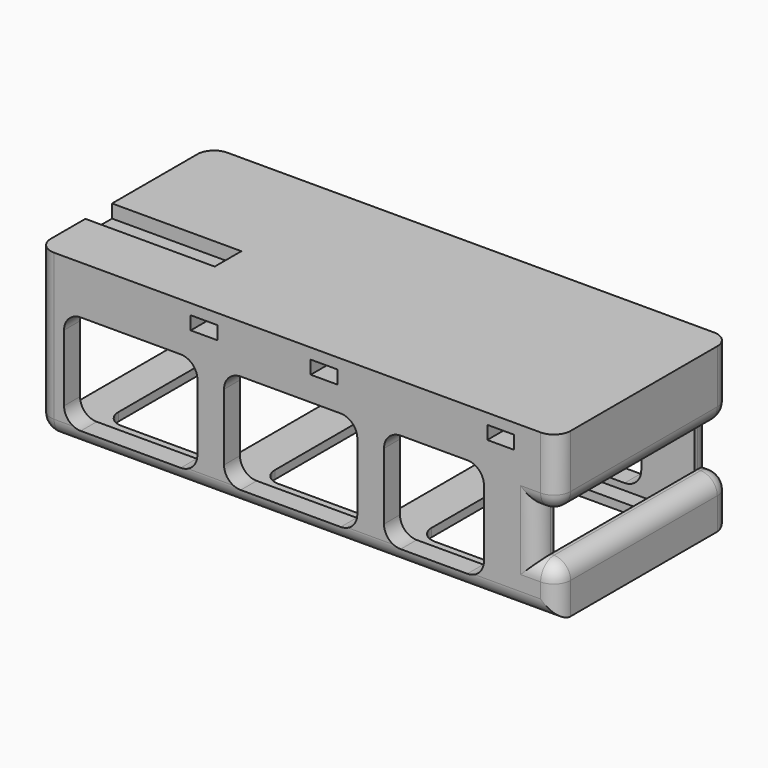
from build123d import *

# Parameters (mm, degrees)
F0_W          = 152
F0_H          = 55
F1_DEPTH      = 39
F2_W          = 53
F2_H          = 34
F3_DEPTH      = 150
F5_DEPTH      = 10.9
F7_DEPTH      = 100
F8_DEPTH      = 5
F9_DEPTH      = 4
F10_DEPTH     = 5
F11_DEPTH     = 5
F12_DEPTH     = 5
F13_W         = 8
F13_H         = 4
F14_DEPTH     = 100
F15_T1_DEPTH  = 163.5
F15_T3_DEPTH  = 74
F15_T5_DEPTH  = 56.5
F15_T7_DEPTH  = 55
F15_S11_W     = 5
F15_S11_H     = 5
F15_T12_DEPTH = 5
F15_S17_W     = 5
F15_S17_H     = 5
F15_T18_DEPTH = 5
F16_W         = 7.2434431314
F16_H         = 13.5
F16_W_2       = 55
F16_W_3       = 10.0454574823
F17_DEPTH     = 6
F18_R         = 5
F19_W         = 10
F19_H         = 4
F20_DEPTH     = 38.8


# Not quite as in the source:
# - a fillet or chamfer that OpenCascade refuses, or shapes differently, is made with other operations: its cross-section is extruded or revolved along the edge and cut away or added


with BuildPart() as f1:
    # F0 (on Top) → F1 (new body)
    with BuildSketch(Plane.XY):
        Rectangle(F0_W, F0_H)
    extrude(amount=F1_DEPTH)

    # F2 (on face) → F3 (cut)
    with BuildSketch(Plane(origin=(-76, 0, 0), x_dir=(0, -1, 0), z_dir=(-1, 0, 0))):
        with Locations((0, 19.5)):
            Rectangle(F2_W, F2_H)
    extrude(amount=-F3_DEPTH, mode=Mode.SUBTRACT)

    # F4 (on face) → F5 (cut)
    with BuildSketch(Plane(origin=(0, 0, 0), x_dir=(1, 0, 0), z_dir=(0, 0, -1))):
        with BuildLine():
            ThreePointArc((-29.5, 16.5), (-30.9644660941, 20.0355339059), (-34.5, 21.5))
            Line((-34.5, 21.5), (-59.5, 21.5))
            ThreePointArc((-59.5, 21.5), (-63.0355339059, 20.0355339059), (-64.5, 16.5))
            Line((-64.5, 16.5), (-64.5, -16.5))
            ThreePointArc((-64.5, -16.5), (-63.0355339059, -20.0355339059), (-59.5, -21.5))
            Line((-59.5, -21.5), (-34.5, -21.5))
            ThreePointArc((-34.5, -21.5), (-30.9644660941, -20.0355339059), (-29.5, -16.5))
            Line((-29.5, -16.5), (-29.5, 16.5))
        make_face()
        with BuildLine():
            Line((-12.5, -21.5), (12.5, -21.5))
            ThreePointArc((12.5, -21.5), (16.0355339059, -20.0355339059), (17.5, -16.5))
            Line((17.5, -16.5), (17.5, 16.5))
            ThreePointArc((17.5, 16.5), (16.0355339059, 20.0355339059), (12.5, 21.5))
            Line((12.5, 21.5), (-12.5, 21.5))
            ThreePointArc((-12.5, 21.5), (-16.0355339059, 20.0355339059), (-17.5, 16.5))
            Line((-17.5, 16.5), (-17.5, -16.5))
            ThreePointArc((-17.5, -16.5), (-16.0355339059, -20.0355339059), (-12.5, -21.5))
        make_face()
        with BuildLine():
            ThreePointArc((64.5, 16.5), (63.0355339059, 20.0355339059), (59.5, 21.5))
            Line((59.5, 21.5), (34.5, 21.5))
            ThreePointArc((34.5, 21.5), (30.9644660941, 20.0355339059), (29.5, 16.5))
            Line((29.5, 16.5), (29.5, -16.5))
            ThreePointArc((29.5, -16.5), (30.9644660941, -20.0355339059), (34.5, -21.5))
            Line((34.5, -21.5), (59.5, -21.5))
            ThreePointArc((59.5, -21.5), (63.0355339059, -20.0355339059), (64.5, -16.5))
            Line((64.5, -16.5), (64.5, 16.5))
        make_face()
    extrude(amount=-F5_DEPTH, mode=Mode.SUBTRACT)

    # F6 (on face) → F7 (cut)
    with BuildSketch(Plane.XZ.offset(27.5)):
        with BuildLine():
            ThreePointArc((-28, 29.5), (-29.4644660941, 33.0355339059), (-33, 34.5))
            Line((-33, 34.5), (-63, 34.5))
            ThreePointArc((-63, 34.5), (-66.5355339059, 33.0355339059), (-68, 29.5))
            Line((-68, 29.5), (-68, 9.5))
            ThreePointArc((-68, 9.5), (-66.5355339059, 5.9644660941), (-63, 4.5))
            Line((-63, 4.5), (-33, 4.5))
            ThreePointArc((-33, 4.5), (-29.4644660941, 5.9644660941), (-28, 9.5))
            Line((-28, 9.5), (-28, 29.5))
        make_face()
        with BuildLine():
            ThreePointArc((20, 29.5), (18.5355339059, 33.0355339059), (15, 34.5))
            Line((15, 34.5), (-15, 34.5))
            ThreePointArc((-15, 34.5), (-18.5355339059, 33.0355339059), (-20, 29.5))
            Line((-20, 29.5), (-20, 9.5))
            ThreePointArc((-20, 9.5), (-18.5355339059, 5.9644660941), (-15, 4.5))
            Line((-15, 4.5), (15, 4.5))
            ThreePointArc((15, 4.5), (18.5355339059, 5.9644660941), (20, 9.5))
            Line((20, 9.5), (20, 29.5))
        make_face()
        with BuildLine():
            ThreePointArc((58, 29.5), (56.5355339059, 33.0355339059), (53, 34.5))
            Line((53, 34.5), (33, 34.5))
            ThreePointArc((33, 34.5), (29.4644660941, 33.0355339059), (28, 29.5))
            Line((28, 29.5), (28, 9.5))
            ThreePointArc((28, 9.5), (29.4644660941, 5.9644660941), (33, 4.5))
            Line((33, 4.5), (53, 4.5))
            ThreePointArc((53, 4.5), (56.5355339059, 5.9644660941), (58, 9.5))
            Line((58, 9.5), (58, 29.5))
        make_face()
    extrude(amount=-F7_DEPTH, mode=Mode.SUBTRACT)

    # F8 (add): a face of the model
    f8_faces = [f1.faces().sort_by_distance(p)[0] for p in [
        (0, 0, 39),
    ]]
    extrude(f8_faces, amount=F8_DEPTH)

    # F9 (add): a face of the model
    f9_faces = [f1.faces().sort_by_distance(p)[0] for p in [
        (76, 0, 22),
    ]]
    extrude(f9_faces, amount=F9_DEPTH)

    # F10 (add): a face of the model
    f10_faces = [f1.faces().sort_by_distance(p)[0] for p in [
        (2, 0, 44),
    ]]
    extrude(f10_faces, amount=F10_DEPTH)

    # F11 (add): a face of the model
    f11_faces = [f1.faces().sort_by_distance(p)[0] for p in [
        (-74.3648547465, 27.5, 24.5),
    ]]
    extrude(f11_faces, amount=F11_DEPTH)

    # F12 (add): a face of the model
    f12_faces = [f1.faces().sort_by_distance(p)[0] for p in [
        (-74.3648547465, -27.5, 24.5),
    ]]
    extrude(f12_faces, amount=F12_DEPTH)

    # F13 (on face) → F14 (cut)
    with BuildSketch(Plane.XZ.offset(32.5)):
        with Locations((-26, 43.8039299548)):
            Rectangle(F13_W, F13_H)
        with Locations((10, 43.8039299548)):
            Rectangle(F13_W, F13_H)
        with Locations((63, 43.8039299548)):
            Rectangle(F13_W, F13_H)
    extrude(amount=-F14_DEPTH, mode=Mode.SUBTRACT)

    # F15: fillet of radius 5 on 7 edges, made by hand

    # F15_s2 → F15_t1 (cut)
    with BuildSketch(Plane.YZ.offset(-71)):
        with BuildLine():
            ThreePointArc((-27.5, 0), (-31.0355339059, 1.4644660941), (-32.5, 5))
            Line((-32.5, 5), (-32.5, 0))
            Line((-32.5, 0), (-27.5, 0))
        make_face()
        with BuildLine():
            ThreePointArc((27.5, 0), (31.0355339059, 1.4644660941), (32.5, 5))
            Line((32.5, 5), (32.5, 0))
            Line((32.5, 0), (27.5, 0))
        make_face()
    extrude(amount=F15_T1_DEPTH, mode=Mode.SUBTRACT)

    # F15_s4 → F15_t3 (cut)
    with BuildSketch(Plane.XY.offset(-12.5)):
        with BuildLine():
            ThreePointArc((80, 27.5), (78.5355339059, 31.0355339059), (75, 32.5))
            Line((75, 32.5), (80, 32.5))
            Line((80, 32.5), (80, 27.5))
        make_face()
        with BuildLine():
            ThreePointArc((80, -27.5), (78.5355339059, -31.0355339059), (75, -32.5))
            Line((75, -32.5), (80, -32.5))
            Line((80, -32.5), (80, -27.5))
        make_face()
    extrude(amount=F15_T3_DEPTH, mode=Mode.SUBTRACT)

    # F15_s6 → F15_t5 (cut)
    with BuildSketch(Plane.XY.offset(5)):
        with BuildLine():
            ThreePointArc((-76, -27.5), (-74.5355339059, -31.0355339059), (-71, -32.5))
            Line((-71, -32.5), (-76, -32.5))
            Line((-76, -32.5), (-76, -27.5))
        make_face()
        with BuildLine():
            ThreePointArc((-71, 32.5), (-74.5355339059, 31.0355339059), (-76, 27.5))
            Line((-76, 27.5), (-76, 32.5))
            Line((-76, 32.5), (-71, 32.5))
        make_face()
    extrude(amount=F15_T5_DEPTH, mode=Mode.SUBTRACT)

    # F15_s8 → F15_t7 (cut)
    with BuildSketch(Plane.XZ.offset(-27.5)):
        with BuildLine():
            ThreePointArc((-71, 0), (-74.5355339059, 1.4644660941), (-76, 5))
            Line((-76, 5), (-76, 0))
            Line((-76, 0), (-71, 0))
        make_face()
    extrude(amount=F15_T7_DEPTH, mode=Mode.SUBTRACT)


with BuildPart() as f15_tool10:
    # F15_s11 → F15_t12 (new body)
    with BuildSketch(Plane.XY.offset(5)):
        with Locations((-73.5, -30)):
            Rectangle(F15_S11_W, F15_S11_H)
    extrude(amount=-F15_T12_DEPTH)

    # F15_s13 → F15_t14 (revolve, cut)
    with BuildSketch(Plane(origin=(-71, -27.5, 5), x_dir=(0.7071067812, 0.7071067812, 0), z_dir=(-0.7071067812, 0.7071067812, 0))):
        with BuildLine():
            ThreePointArc((0, -5), (5, 0), (0, 5))
            Line((0, 5), (0, -5))
        make_face()
    revolve(axis=Axis((-71, -27.5, 5), (0, 0, -1)), mode=Mode.SUBTRACT)


with BuildPart() as f1_1:
    add(f1.part)

    # F15_t9: cut F15_tool10
    add(f15_tool10.part, mode=Mode.SUBTRACT)


with BuildPart() as f15_tool16:
    # F15_s17 → F15_t18 (new body)
    with BuildSketch(Plane.XY.offset(5)):
        with Locations((-73.5, 30)):
            Rectangle(F15_S17_W, F15_S17_H)
    extrude(amount=-F15_T18_DEPTH)

    # F15_s19 → F15_t20 (revolve, cut)
    with BuildSketch(Plane(origin=(-71, 27.5, 5), x_dir=(0.7071067812, -0.7071067812, 0), z_dir=(0.7071067812, 0.7071067812, 0))):
        with BuildLine():
            ThreePointArc((0, -5), (5, 0), (0, 5))
            Line((0, 5), (0, -5))
        make_face()
    revolve(axis=Axis((-71, 27.5, 5), (0, 0, -1)), mode=Mode.SUBTRACT)


with BuildPart() as f1_2:
    add(f1_1.part)

    # F15_t15: cut F15_tool16
    add(f15_tool16.part, mode=Mode.SUBTRACT)

    # F16 (on face) → F17 (cut)
    with BuildSketch(Plane.YZ.offset(80)):
        with Locations((-31.1217215657, 21.25)):
            Rectangle(F16_W, F16_H)
        with Locations((0, 21.25)):
            Rectangle(F16_W_2, F16_H)
        with Locations((32.5227287412, 21.25)):
            Rectangle(F16_W_3, F16_H)
    extrude(amount=-F17_DEPTH, mode=Mode.SUBTRACT)

    # F18
    f18_edges = [f1_2.edges().sort_by_distance(p)[0] for p in [
        (74, -32.5, 21.25),
        (74, 32.5, 21.25),
        (80, 0, 28),
        (80, 0, 14.5),
    ]]
    fillet(f18_edges, radius=F18_R)

    # F19 (on face) → F20 (cut)
    with BuildSketch(Plane(origin=(-76, 0, 0), x_dir=(0, -1, 0), z_dir=(-1, 0, 0))):
        with Locations((9.5, 47)):
            Rectangle(F19_W, F19_H)
    extrude(amount=-F20_DEPTH, mode=Mode.SUBTRACT)


solid = f1_2.part
